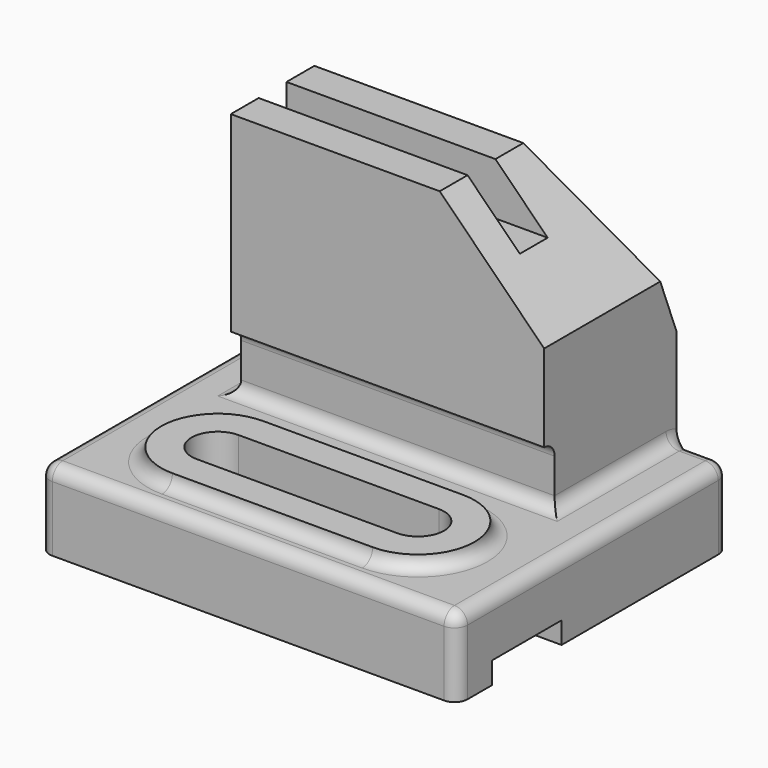
from build123d import *

# Parameters (mm, degrees)
F0_W          = 96
F0_H          = 78
F1_DEPTH      = 18
F2_W          = 72
F2_H          = 38
F3_DEPTH      = 58
F4_R          = 3
F5_W          = 72
F5_H          = 8
F6_DEPTH      = 12
F7_C1_SIZE    = 24
F8_SIZE2      = 14
F8_SIZE       = 36
F9_W          = 3
F9_H          = 14
F10_DEPTH     = 72
F11_W         = 20
F11_H         = 5
F12_DEPTH     = 96
F14_DEPTH     = 3
F16_DEPTH     = 16
F17_T1_DEPTH  = 72
F17_T3_DEPTH  = 32
F17_T5_DEPTH  = 46
F17_T8_ANGLE  = 180
F17_T10_ANGLE = 180
F17_T14_ANGLE = 233.2969892374
F17_T19_ANGLE = 233.2969892374
F17_T25_DEPTH = 39.5
F17_T29_DEPTH = 79.5
F17_T36_DEPTH = 79.5
F17_T40_DEPTH = 39.5
F17_T43_DEPTH = 22.5
F17_T45_DEPTH = 90
F17_T47_DEPTH = 72
F17_S51_W     = 3.06
F17_S51_H     = 3.06
F17_T52_DEPTH = 3.06
F17_S57_W     = 3.06
F17_S57_H     = 3.06
F17_T58_DEPTH = 3.06
F17_T62_ANGLE = 90
F17_T64_ANGLE = 90


# Not quite as in the source:
# - a fillet or chamfer that OpenCascade refuses, or shapes differently, is made with other operations: its cross-section is extruded or revolved along the edge and cut away or added


with BuildPart() as f1:
    # F0 (on Top) → F1 (new body)
    with BuildSketch(Plane.XY):
        with Locations((48, 39)):
            Rectangle(F0_W, F0_H)
    extrude(amount=F1_DEPTH)

    # F2 (on face) → F3 (join)
    with BuildSketch(Plane.XY.offset(18)):
        with Locations((48, 59)):
            Rectangle(F2_W, F2_H)
    extrude(amount=F3_DEPTH)

    # F4
    f4_edges = [f1.edges().sort_by_distance(p)[0] for p in [
        (90, 78, 18),
        (6, 78, 18),
    ]]
    fillet(f4_edges, radius=F4_R)

    # F5 (on face) → F6 (cut)
    with BuildSketch(Plane.XY.offset(76)):
        with Locations((48, 52)):
            Rectangle(F5_W, F5_H)
    extrude(amount=-F6_DEPTH, mode=Mode.SUBTRACT)

    # F7: chamfer of 24 on 2 edges, made by hand

    # F7_c1
    f7_c1_edges = [f1.edges().sort_by_distance(p)[0] for p in [
        (84, 44, 76),
    ]]
    chamfer(f7_c1_edges, length=F7_C1_SIZE)

    # F8
    f8_edges = [f1.edges().sort_by_distance(p)[0] for p in [
        (36, 78, 76),
    ]]
    f8_side = f1.faces().sort_by_distance((46.545455, 78, 34.461039))[0]
    chamfer(f8_edges, length=F8_SIZE, length2=F8_SIZE2, reference=f8_side)

    # F9 (on face) → F10 (cut, through all)
    with BuildSketch(Plane.YZ.offset(84)):
        with Locations((41.5, 25)):
            Rectangle(F9_W, F9_H)
    extrude(amount=-F10_DEPTH, mode=Mode.SUBTRACT)

    # F11 (on face) → F12 (cut, through all)
    with BuildSketch(Plane.YZ.offset(96)):
        with Locations((20, 2.5)):
            Rectangle(F11_W, F11_H)
    extrude(amount=-F12_DEPTH, mode=Mode.SUBTRACT)

    # F13 (on face) → F14 (join)
    with BuildSketch(Plane.XY.offset(18)):
        with BuildLine():
            ThreePointArc((71, 7), (84, 20), (71, 33))
            Line((71, 33), (25, 33))
            ThreePointArc((25, 33), (12, 20), (25, 7))
            Line((25, 7), (71, 7))
        make_face()
    extrude(amount=F14_DEPTH)

    # F15 (on face) → F16 (cut, through all)
    with BuildSketch(Plane.XY.offset(21)):
        with BuildLine():
            ThreePointArc((25, 26), (19, 20), (25, 14))
            Line((25, 14), (71, 14))
            ThreePointArc((71, 14), (77, 20), (71, 26))
            Line((71, 26), (25, 26))
        make_face()
    extrude(amount=-F16_DEPTH, mode=Mode.SUBTRACT)

    # F17: fillet of radius 3 on 17 edges, made by hand

    # F17_s2 → F17_t1 (join)
    with BuildSketch(Plane.YZ.offset(12)):
        with BuildLine():
            ThreePointArc((40, 32), (42.1213203436, 31.1213203436), (43, 29))
            Line((43, 29), (43, 32))
            Line((43, 32), (40, 32))
        make_face()
        with BuildLine():
            ThreePointArc((43, 21), (42.1213203436, 18.8786796564), (40, 18))
            Line((40, 18), (43, 18))
            Line((43, 18), (43, 21))
        make_face()
    extrude(amount=F17_T1_DEPTH)

    # F17_s4 → F17_t3 (join)
    with BuildSketch(Plane.XZ.offset(-75)):
        with BuildLine():
            ThreePointArc((84, 21), (84.8786796564, 18.8786796564), (87, 18))
            Line((87, 18), (84, 18))
            Line((84, 18), (84, 21))
        make_face()
        with BuildLine():
            ThreePointArc((9, 18), (11.1213203436, 18.8786796564), (12, 21))
            Line((12, 21), (12, 18))
            Line((12, 18), (9, 18))
        make_face()
    extrude(amount=F17_T3_DEPTH)

    # F17_s6 → F17_t5 (join)
    with BuildSketch(Plane.YZ.offset(25)):
        with BuildLine():
            ThreePointArc((4, 18), (6.1213203436, 18.8786796564), (7, 21))
            Line((7, 21), (7, 18))
            Line((7, 18), (4, 18))
        make_face()
        with BuildLine():
            ThreePointArc((36, 18), (33.8786796564, 18.8786796564), (33, 21))
            Line((33, 21), (33, 18))
            Line((33, 18), (36, 18))
        make_face()
    extrude(amount=F17_T5_DEPTH)

    # F17_s7 → F17_t8 (revolve)
    with BuildSketch(Plane.YZ.offset(25)):
        with BuildLine():
            ThreePointArc((36, 18), (33.8786796564, 18.8786796564), (33, 21))
            Line((33, 21), (33, 18))
            Line((33, 18), (36, 18))
        make_face()
    revolve(axis=Axis((25, 20, 18), (0, 0, 1)), revolution_arc=F17_T8_ANGLE)

    # F17_s9 → F17_t10 (revolve)
    with BuildSketch(Plane.YZ.offset(71)):
        with BuildLine():
            ThreePointArc((4, 18), (6.1213203436, 18.8786796564), (7, 21))
            Line((7, 21), (7, 18))
            Line((7, 18), (4, 18))
        make_face()
    revolve(axis=Axis((71, 20, 18), (0, 0, 1)), revolution_arc=F17_T10_ANGLE)


with BuildPart() as f17_tool12:
    # F17_s13 → F17_t14 (revolve)
    with BuildSketch(Plane(origin=(0, 19.6028186536, -26.2963148857), x_dir=(1, 0, 0), z_dir=(0, -0.5976672776, 0.8017442393))):
        with BuildLine():
            ThreePointArc((12, 63.0958271118), (11.1213203436, 65.2171474554), (9, 66.0958271118))
            Line((9, 66.0958271118), (12, 66.0958271118))
            Line((12, 66.0958271118), (12, 63.0958271118))
        make_face()
    revolve(axis=Axis((12, 75, 15), (1, 0, 0)), revolution_arc=F17_T14_ANGLE)

    split(bisect_by=Plane.XZ.offset(-78), keep=Keep.TOP)


with BuildPart() as f1_1:
    add(f1.part)

    # F17_t11: union F17_tool12
    add(f17_tool12.part)


with BuildPart() as f17_tool17:
    # F17_s18 → F17_t19 (revolve)
    with BuildSketch(Plane(origin=(0, 19.6028186536, -26.2963148857), x_dir=(1, 0, 0), z_dir=(0, -0.5976672776, 0.8017442393))):
        with BuildLine():
            ThreePointArc((84, 63.0958271118), (84.8786796564, 65.2171474554), (87, 66.0958271118))
            Line((87, 66.0958271118), (84, 66.0958271118))
            Line((84, 66.0958271118), (84, 63.0958271118))
        make_face()
    revolve(axis=Axis((84, 75, 15), (1, 0, 0)), revolution_arc=F17_T19_ANGLE)

    split(bisect_by=Plane.XZ.offset(-78), keep=Keep.TOP)


with BuildPart() as f1_2:
    add(f1_1.part)

    # F17_t16: union F17_tool17
    add(f17_tool17.part)


with BuildPart() as f17_tool23:
    # F17_s24 → F17_t25 (new body)
    with BuildSketch(Plane.XZ.offset(-35.5)):
        with BuildLine():
            ThreePointArc((84, 21), (84.8786796564, 18.8786796564), (87, 18))
            Line((87, 18), (84, 18))
            Line((84, 18), (84, 21))
        make_face()
    extrude(amount=-F17_T25_DEPTH)

    split(bisect_by=Plane.XZ.offset(-43), keep=Keep.TOP)


with BuildPart() as f17_tool27:
    # F17_s28 → F17_t29 (new body)
    with BuildSketch(Plane.YZ.offset(91.5)):
        with BuildLine():
            ThreePointArc((43, 21), (42.1213203436, 18.8786796564), (40, 18))
            Line((40, 18), (43, 18))
            Line((43, 18), (43, 21))
        make_face()
    extrude(amount=-F17_T29_DEPTH)

    split(bisect_by=Plane.YZ.offset(84), keep=Keep.TOP)


with BuildPart() as f17_tool23_1:
    add(f17_tool23.part)

    # F17_t31: intersect F17_tool27
    add(f17_tool27.part, mode=Mode.INTERSECT)


with BuildPart() as f1_3:
    add(f1_2.part)

    # F17_t21: union F17_tool23
    add(f17_tool23_1.part)


with BuildPart() as f17_tool34:
    # F17_s35 → F17_t36 (new body)
    with BuildSketch(Plane.YZ.offset(84)):
        with BuildLine():
            ThreePointArc((43, 21), (42.1213203436, 18.8786796564), (40, 18))
            Line((40, 18), (43, 18))
            Line((43, 18), (43, 21))
        make_face()
    extrude(amount=-F17_T36_DEPTH)

    split(bisect_by=Plane.YZ.offset(12), keep=Keep.BOTTOM)


with BuildPart() as f17_tool38:
    # F17_s39 → F17_t40 (new body)
    with BuildSketch(Plane.XZ.offset(-75)):
        with BuildLine():
            ThreePointArc((9, 18), (11.1213203436, 18.8786796564), (12, 21))
            Line((12, 21), (12, 18))
            Line((12, 18), (9, 18))
        make_face()
    extrude(amount=F17_T40_DEPTH)

    split(bisect_by=Plane.XZ.offset(-43), keep=Keep.TOP)


with BuildPart() as f17_tool34_1:
    add(f17_tool34.part)

    # F17_t42: intersect F17_tool38
    add(f17_tool38.part, mode=Mode.INTERSECT)


with BuildPart() as f1_4:
    add(f1_3.part)

    # F17_t32: union F17_tool34
    add(f17_tool34_1.part)

    # F17_s44 → F17_t43 (cut)
    with BuildSketch(Plane.XY.offset(-7.5)):
        with BuildLine():
            ThreePointArc((3, 0), (0.8786796564, 0.8786796564), (0, 3))
            Line((0, 3), (0, 0))
            Line((0, 0), (3, 0))
        make_face()
        with BuildLine():
            ThreePointArc((96, 3), (95.1213203436, 0.8786796564), (93, 0))
            Line((93, 0), (96, 0))
            Line((96, 0), (96, 3))
        make_face()
        with BuildLine():
            ThreePointArc((0, 75), (0.8786796564, 77.1213203436), (3, 78))
            Line((3, 78), (0, 78))
            Line((0, 78), (0, 75))
        make_face()
        with BuildLine():
            ThreePointArc((96, 75), (95.1213203436, 77.1213203436), (93, 78))
            Line((93, 78), (96, 78))
            Line((96, 78), (96, 75))
        make_face()
    extrude(amount=F17_T43_DEPTH, mode=Mode.SUBTRACT)

    # F17_s46 → F17_t45 (cut)
    with BuildSketch(Plane.YZ.offset(3)):
        with BuildLine():
            ThreePointArc((3, 18), (0.8786796564, 17.1213203436), (0, 15))
            Line((0, 15), (0, 18))
            Line((0, 18), (3, 18))
        make_face()
    extrude(amount=F17_T45_DEPTH, mode=Mode.SUBTRACT)

    # F17_s48 → F17_t47 (cut)
    with BuildSketch(Plane.XZ.offset(-75)):
        with BuildLine():
            ThreePointArc((3, 18), (0.8786796564, 17.1213203436), (0, 15))
            Line((0, 15), (0, 18))
            Line((0, 18), (3, 18))
        make_face()
        with BuildLine():
            ThreePointArc((93, 18), (95.1213203436, 17.1213203436), (96, 15))
            Line((96, 15), (96, 18))
            Line((96, 18), (93, 18))
        make_face()
    extrude(amount=F17_T47_DEPTH, mode=Mode.SUBTRACT)


with BuildPart() as f17_tool50:
    # F17_s51 → F17_t52 (new body)
    with BuildSketch(Plane.XY.offset(15)):
        with Locations((1.47, 1.47)):
            Rectangle(F17_S51_W, F17_S51_H)
    extrude(amount=F17_T52_DEPTH)

    # F17_s53 → F17_t54 (revolve, cut)
    with BuildSketch(Plane(origin=(3, 3, 15), x_dir=(0.7071067812, 0.7071067812, 0), z_dir=(0.7071067812, -0.7071067812, 0))):
        with BuildLine():
            ThreePointArc((0, -3), (3, 0), (0, 3))
            Line((0, 3), (0, -3))
        make_face()
    revolve(axis=Axis((3, 3, 15), (0, 0, 1)), mode=Mode.SUBTRACT)


with BuildPart() as f1_5:
    add(f1_4.part)

    # F17_t49: cut F17_tool50
    add(f17_tool50.part, mode=Mode.SUBTRACT)


with BuildPart() as f17_tool56:
    # F17_s57 → F17_t58 (new body)
    with BuildSketch(Plane.YZ.offset(93)):
        with Locations((1.47, 16.53)):
            Rectangle(F17_S57_W, F17_S57_H)
    extrude(amount=F17_T58_DEPTH)

    # F17_s59 → F17_t60 (revolve, cut)
    with BuildSketch(Plane(origin=(93, 3, 15), x_dir=(0, 0.7071067812, -0.7071067812), z_dir=(0, -0.7071067812, -0.7071067812))):
        with BuildLine():
            ThreePointArc((0, -3), (3, 0), (0, 3))
            Line((0, 3), (0, -3))
        make_face()
    revolve(axis=Axis((93, 3, 15), (1, 0, 0)), mode=Mode.SUBTRACT)


with BuildPart() as f1_6:
    add(f1_5.part)

    # F17_t55: cut F17_tool56
    add(f17_tool56.part, mode=Mode.SUBTRACT)

    # F17_s61 → F17_t62 (revolve, cut)
    with BuildSketch(Plane.XY.offset(15)):
        with BuildLine():
            ThreePointArc((93, 78), (95.1213203436, 77.1213203436), (96, 75))
            Line((96, 75), (96, 78))
            Line((96, 78), (93, 78))
        make_face()
    revolve(axis=Axis((96, 75, 15), (1, 0, 0)), revolution_arc=F17_T62_ANGLE, mode=Mode.SUBTRACT)

    # F17_s63 → F17_t64 (revolve, cut)
    with BuildSketch(Plane.XY.offset(15)):
        with BuildLine():
            ThreePointArc((0, 75), (0.8786796564, 77.1213203436), (3, 78))
            Line((3, 78), (0, 78))
            Line((0, 78), (0, 75))
        make_face()
    revolve(axis=Axis((0, 75, 15), (1, 0, 0)), revolution_arc=F17_T64_ANGLE, mode=Mode.SUBTRACT)


solid = f1_6.part
